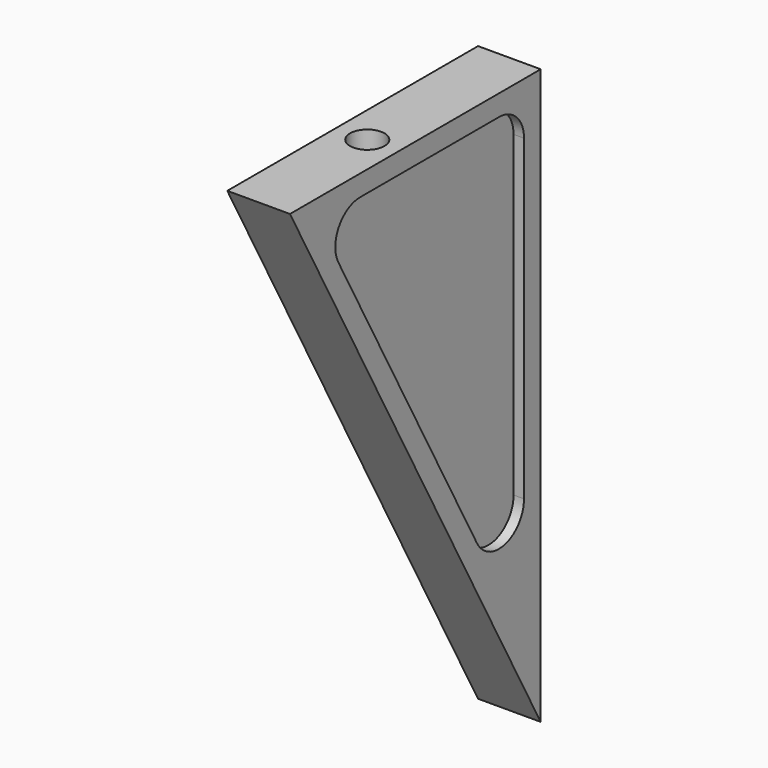
from build123d import *

# Parameters (mm, degrees)
F1_DEPTH = 3
F3_D     = 3.3
F3_DEPTH = 10
F3_TIP   = 0.9914200214
F5_D     = 3.3
F5_DEPTH = 12
F5_TIP   = 0.9914200214
F7_DEPTH = 1


# Not quite as in the source:
# - a pattern or mirror of a feature is missing from the dataset's text; its kind, count and spacing are read off the source's solid
# - a feature names something its author has since deleted; it is built from what else it names


with BuildPart() as f1:
    # F0 (on Right) → F1 (new body, symmetric)
    with BuildSketch(Plane.YZ):
        Polygon((0, -55), (0, 0), (-30, 0), align=None)
    extrude(amount=F1_DEPTH, both=True)

    # F3
    with Locations(Plane(origin=(0, 0, 0), x_dir=(-1, 0, 0), z_dir=(0, 1, 0))):
        with Locations((0, -10), (0, -30)):
            Hole(F3_D / 2, depth=F3_DEPTH)
            with Locations((0, 0, -(F3_DEPTH + F3_TIP / 2))):  # 118° drill point
                Cone(0, F3_D / 2, F3_TIP, mode=Mode.SUBTRACT)

    # F5
    with Locations(Plane.XY):
        with Locations((0, -17)):
            Hole(F5_D / 2, depth=F5_DEPTH)
            with Locations((0, 0, -(F5_DEPTH + F5_TIP / 2))):  # 118° drill point
                Cone(0, F5_D / 2, F5_TIP, mode=Mode.SUBTRACT)

    # F6 (on face) → F7 (cut)
    with BuildSketch(Plane.YZ.offset(3)):
        with BuildLine():
            ThreePointArc((-2, -5), (-2.8786796564, -2.8786796564), (-5, -2))
            Line((-5, -2), (-21.5772890518, -2))
            ThreePointArc((-21.5772890518, -2), (-24.1569856595, -3.4686067089), (-24.2109757705, -6.436556392))
            Line((-24.2109757705, -6.436556392), (-7.6336867187, -36.8282529869))
            ThreePointArc((-7.6336867187, -36.8282529869), (-4.258737616, -38.2986761404), (-2, -35.3916965949))
            Line((-2, -35.3916965949), (-2, -5))
        make_face()
    f7 = extrude(amount=-F7_DEPTH, mode=Mode.SUBTRACT)

    # F7_copies: F7 across plane
    add(f7.mirror(Plane(origin=(0, 0, 0), x_dir=(0, 0, -1), z_dir=(-1, 0, 0))), mode=Mode.SUBTRACT)


solid = f1.part
